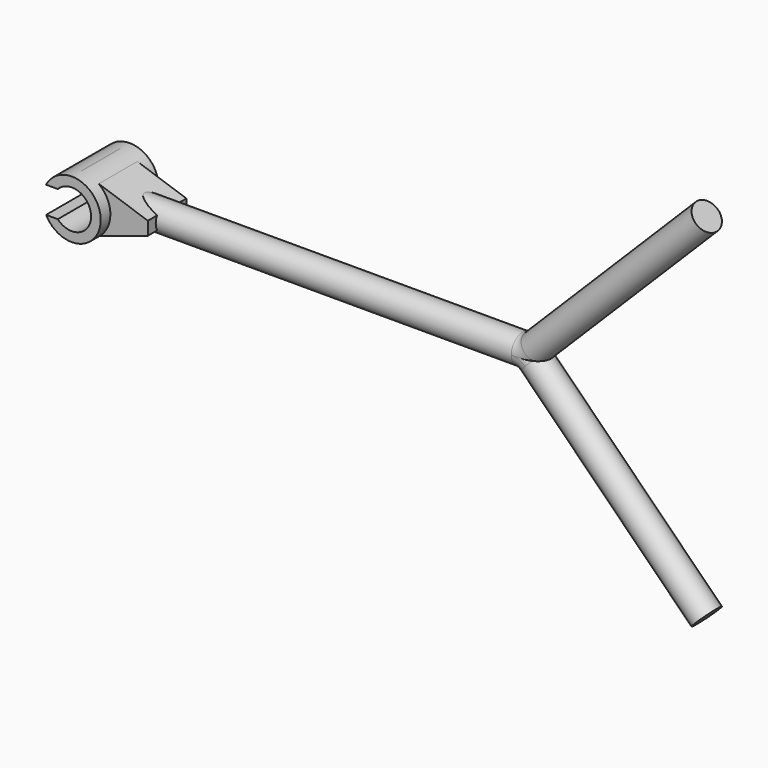
from build123d import *

# Parameters (mm, degrees)
F0_R             = 6
F0_R_2           = 4
F1_DEPTH         = 7.5
F3_R             = 2.95
F4_DEPTH         = 80
F5_W             = 20
F5_H             = 5.5
F6_DEPTH         = 25
F12_DEPTH        = 5
F14_R            = 2.95
F16_COPIES_COUNT = 2


# Not quite as in the source:
# - a feature of the source that left no trace in its solid (it failed there, or was rolled back) is left out
# - a pattern or mirror of a feature is missing from the dataset's text; its kind, count and spacing are read off the source's solid


with BuildPart() as f1:
    # F0 (on Front) → F1 (new body, symmetric)
    with BuildSketch(Plane.XZ):
        Circle(F0_R)
        Circle(F0_R_2, mode=Mode.SUBTRACT)
    extrude(amount=F1_DEPTH, both=True)

    # F3 (on offset) → F4 (join)
    with BuildSketch(Plane.YZ.offset(4.5)):
        Circle(F3_R)
    extrude(amount=F4_DEPTH)

    # F5 (on face) → F6 (cut)
    with BuildSketch(Plane.XZ.offset(7.5)):
        with Locations((-10, 0)):
            Rectangle(F5_W, F5_H)
    extrude(amount=-F6_DEPTH, mode=Mode.SUBTRACT)

    # F11 (on face) → F12 (join, symmetric)
    with BuildSketch(Plane.XZ):
        Polygon((13.7702096254, 1.3738754205), (0, 6.0186968185), (5.8568101376, 0), (0, -5.9087458067), (13.7702096254, -1.3786113122), align=None)
    extrude(amount=F12_DEPTH, both=True)

    # F16: sweep along a path in F15
    with BuildLine(Plane.XZ) as f16_path:
        Line((84.5, 0), (87.5, 0))
        ThreePointArc((87.5, 0), (89.0307337295, 0.30448187), (90.3284271247, 1.1715728753))
        Line((90.3284271247, 1.1715728753), (125.6837661841, 36.5269119346))
    # F14 (on face) → F16 (sweep)
    with BuildSketch(Plane.YZ.offset(84.5)):
        Circle(F14_R)
    f16 = sweep(path=f16_path.line)

    # F16_copies: F16 ×2 about axis
    f16_copies_axis = Axis((0, 0, 0), (1, 0, 0))
    for i in range(1, F16_COPIES_COUNT):
        add(f16.rotate(f16_copies_axis, i * 360 / F16_COPIES_COUNT))


solid = f1.part
